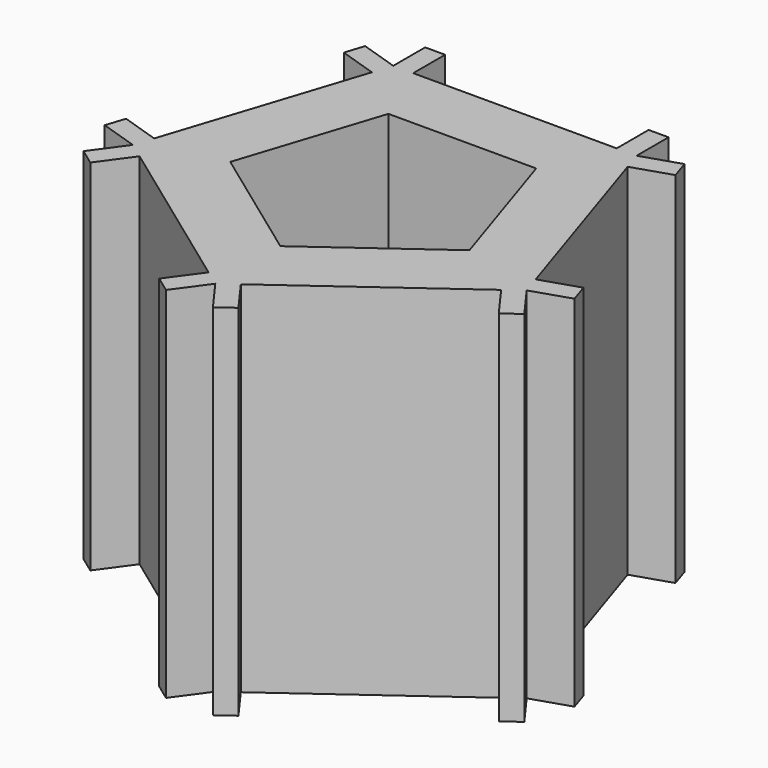
from build123d import *

# Parameters (mm, degrees)
F1_DEPTH  = 18
F2_W      = 1
F2_H      = 18
F3_DEPTH  = 2
F4_W      = 1
F4_H      = 18
F5_DEPTH  = 2
F6_W      = 1
F6_H      = 18
F7_DEPTH  = 2
F8_W      = 1
F8_H      = 18
F9_DEPTH  = 2
F10_W     = 1
F10_H     = 18
F11_DEPTH = 2


with BuildPart() as f1:
    # F0 (on Top) → F1 (new body)
    with BuildSketch(Plane.XY):
        Polygon((0, -10.3779398619), (9.8700073314, -3.2069597839), (6.1, 8.3959297149), (-6.1, 8.3959297149), (-9.8700073314, -3.2069597839), align=None)
        Polygon((-5.9933346782, -1.947352483), (-3.7040845371, 5.0982349887), (3.7040845371, 5.0982349887), (5.9933346782, -1.947352483), (0, -6.3017650113), align=None, mode=Mode.SUBTRACT)
    extrude(amount=F1_DEPTH)

    # F2 (on face) → F3 (join)
    with BuildSketch(Plane(origin=(4.9350036657, -6.7924498229, 0), x_dir=(0.8090169944, 0.5877852523, 0), z_dir=(0.5877852523, -0.8090169944, 0))):
        with Locations((-5.6, 9)):
            Rectangle(F2_W, F2_H)
        with Locations((5.6, 9)):
            Rectangle(F2_W, F2_H)
    extrude(amount=F3_DEPTH)

    # F4 (on face) → F5 (join)
    with BuildSketch(Plane(origin=(-4.9350036657, -6.7924498229, 0), x_dir=(0.8090169944, -0.5877852523, 0), z_dir=(-0.5877852523, -0.8090169944, 0))):
        with Locations((5.6, 9)):
            Rectangle(F4_W, F4_H)
        with Locations((-5.6, 9)):
            Rectangle(F4_W, F4_H)
    extrude(amount=F5_DEPTH)

    # F6 (on face) → F7 (join)
    with BuildSketch(Plane(origin=(-7.9850036657, 2.5944849655, 0), x_dir=(-0.3090169944, -0.9510565163, 0), z_dir=(-0.9510565163, 0.3090169944, 0))):
        with Locations((5.6, 9)):
            Rectangle(F6_W, F6_H)
        with Locations((-5.6, 9)):
            Rectangle(F6_W, F6_H)
    extrude(amount=F7_DEPTH)

    # F8 (on face) → F9 (join)
    with BuildSketch(Plane(origin=(7.9850036657, 2.5944849655, 0), x_dir=(-0.3090169944, 0.9510565163, 0), z_dir=(0.9510565163, 0.3090169944, 0))):
        with Locations((-5.6, 9)):
            Rectangle(F8_W, F8_H)
        with Locations((5.6, 9)):
            Rectangle(F8_W, F8_H)
    extrude(amount=F9_DEPTH)

    # F10 (on face) → F11 (join)
    with BuildSketch(Plane(origin=(0, 8.3959297149, 0), x_dir=(-1, 0, 0), z_dir=(0, 1, 0))):
        with Locations((5.6, 9)):
            Rectangle(F10_W, F10_H)
        with Locations((-5.6, 9)):
            Rectangle(F10_W, F10_H)
    extrude(amount=F11_DEPTH)


solid = f1.part
